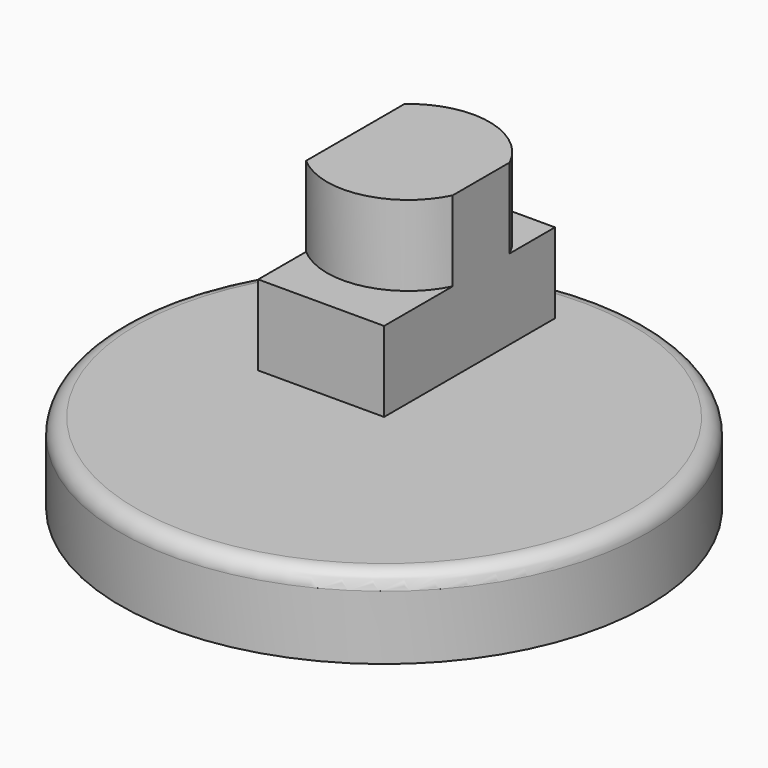
from build123d import *

# Parameters (mm, degrees)
F0_R     = 83.6782279658
F9_DEPTH = 25.4
F1_R     = 5.08
F4_W     = 39.921930186
F4_H     = 67.7046595855
F5_DEPTH = 25.4
F7_DEPTH = 25.4


# Not quite as in the source:
# - a feature of the source that left no trace in its solid (it failed there, or was rolled back) is left out


with BuildPart() as f9:
    # F0 (on Top) → F9 (new body)
    with BuildSketch(Plane.XY):
        with Locations((-32.2435125709, 104.3095961213)):
            Circle(F0_R)
    extrude(amount=F9_DEPTH)

    # F1
    f1_edges = [f9.edges().sort_by_distance(p)[0] for p in [
        (-115.921741, 104.309596, 25.4),
    ]]
    fillet(f1_edges, radius=F1_R)

    # F4 (on face) → F5 (join)
    with BuildSketch(Plane.XY.offset(25.4)):
        with Locations((-52.2044776638, 138.1619259141)):
            Rectangle(F4_W, F4_H)
    extrude(amount=F5_DEPTH)

    # F6 (on face) → F7 (join)
    with BuildSketch(Plane.XY.offset(50.8)):
        with BuildLine():
            Line((-32.2435125709, 131.4756200401), (-32.2435125709, 154.0904118927))
            ThreePointArc((-32.2435125709, 154.0904118927), (-50.1885900091, 168.000528459), (-72.1654427568, 162.2965745269))
            Line((-72.1654427568, 162.2965745269), (-72.1654427568, 123.2694574059))
            ThreePointArc((-72.1654427568, 123.2694574059), (-50.1885900091, 117.5655034739), (-32.2435125709, 131.4756200401))
        make_face()
    extrude(amount=F7_DEPTH)


solid = f9.part
